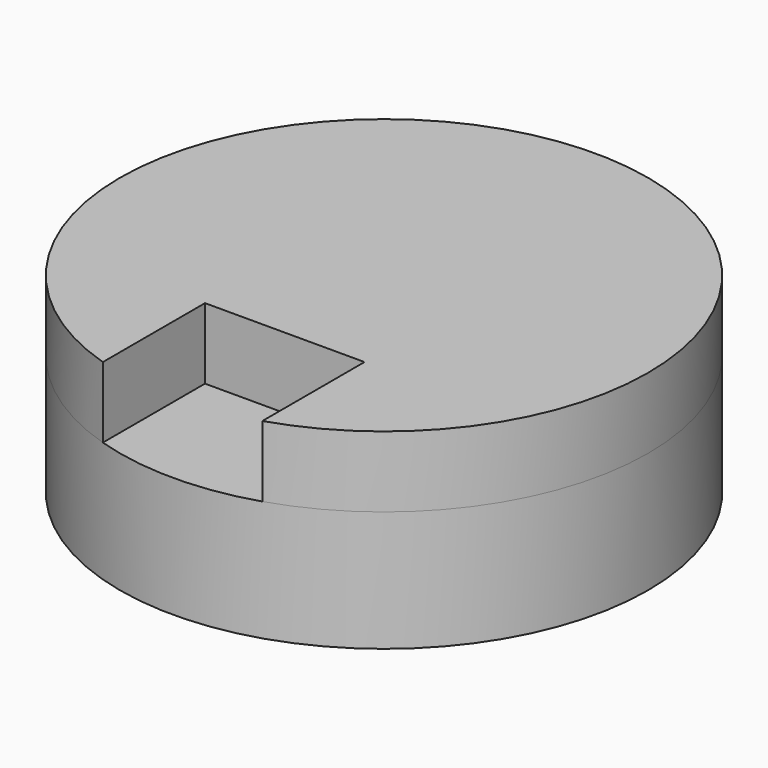
from build123d import *
from build123d import SkipClean  # not in build123d's __all__

# Parameters (mm, degrees)
F1_R     = 7.45
F2_DEPTH = 3.4
F3_DEPTH = 2


with BuildPart() as f2:
    # F1 (on Top) → F2 (new body)
    with BuildSketch(Plane.XY):
        Circle(F1_R)
    extrude(amount=-F2_DEPTH)

    # F0 (on Top) → F3 (join)
    with BuildSketch(Plane.XY):
        with BuildLine():
            Line((2.25, -6.5), (2.25, -7.1021123618))
            ThreePointArc((2.25, -7.1021123618), (0, 7.45), (-2.25, -7.1021123618))
            Line((-2.25, -7.1021123618), (-2.25, -6.5))
            Line((-2.25, -6.5), (-2.25, -3.5))
            Line((-2.25, -3.5), (2.25, -3.5))
            Line((2.25, -3.5), (2.25, -6.5))
        make_face()
    with SkipClean():  # cleaning this boolean's faces spoils the solid; the shape is the same uncleaned
        extrude(amount=F3_DEPTH)


solid = f2.part
